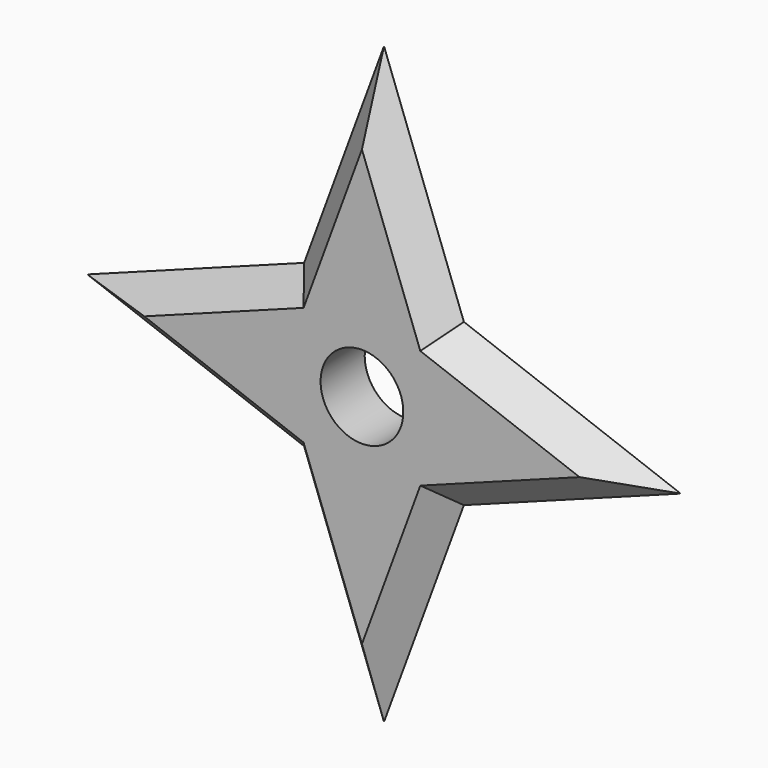
from build123d import *

# Parameters (mm, degrees)
F1_DEPTH = 10.16
F2_SIZE  = 5.07999
F4_D     = 15.24


# Not quite as in the source:
# - a fillet or chamfer is up to 0.001 mm smaller than in the source, because OpenCascade refuses the exact size


with BuildPart() as f1:
    # F0 (on Front) → F1 (new body)
    with BuildSketch(Plane.XZ):
        Polygon((14.7110316902, 14.8611441255), (0, 54.7910891473), (-14.7110316902, 14.8611441255), (0, 0), align=None)
        Polygon((54.6409785748, 0), (14.7110316902, 14.8611441255), (0, 0), (14.7110316902, -14.8611441255), align=None)
        Polygon((14.7110316902, -14.8611441255), (0, 0), (-14.7110316902, -14.8611441255), (0, -54.7910891473), align=None)
        Polygon((0, 0), (-14.7110316902, 14.8611441255), (-54.6409785748, 0), (-14.7110316902, -14.8611441255), align=None)
    extrude(amount=F1_DEPTH)

    # F2 (size 5.08 in the source; OpenCascade refuses exactly that, so slightly less here)
    f2_edges = [f1.edges().sort_by_distance(p)[0] for p in [
        (7.355516, 0, 34.826117),
        (-7.355516, 0, 34.826117),
        (-7.355516, -10.16, 34.826117),
        (7.355516, -10.16, 34.826117),
        (-34.676005, -10.16, 7.430572),
        (-34.676005, 0, 7.430572),
        (-34.676005, -10.16, -7.430572),
        (-34.676005, 0, -7.430572),
        (34.676005, 0, -7.430572),
        (34.676005, 0, 7.430572),
        (34.676005, -10.16, 7.430572),
        (34.676005, -10.16, -7.430572),
        (-7.355516, 0, -34.826117),
        (7.355516, 0, -34.826117),
        (-7.355516, -10.16, -34.826117),
        (7.355516, -10.16, -34.826117),
    ]]
    chamfer(f2_edges, length=F2_SIZE)

    # F4 (through all)
    with Locations(Plane(origin=(0, 0, 0), x_dir=(1, 0, 0), z_dir=(0, 1, 0))):
        with Locations((0, 0)):
            Hole(F4_D / 2)


solid = f1.part
